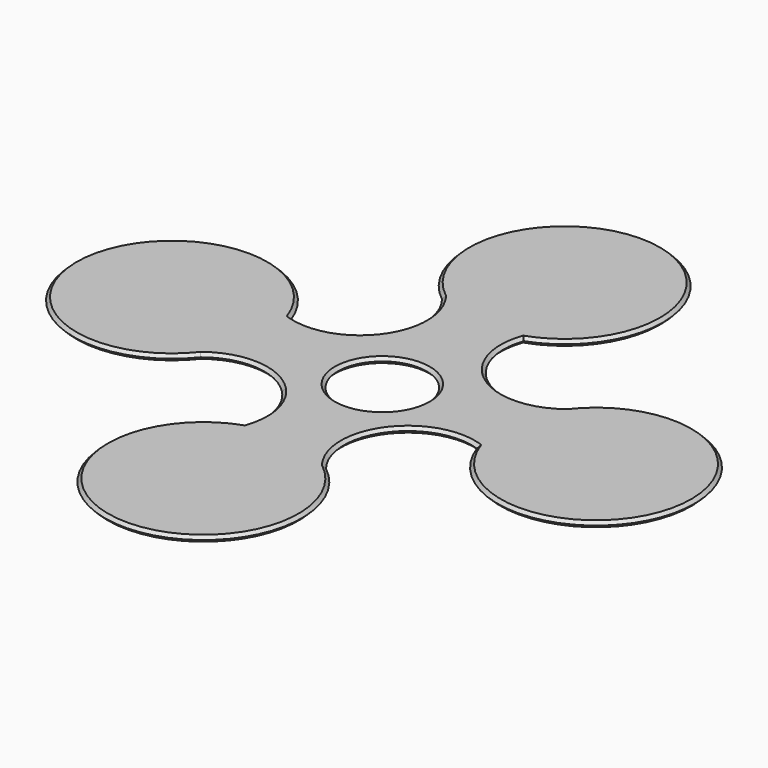
from build123d import *

# Parameters (mm, degrees)
F0_R        = 3.6516934022
F1_DEPTH    = 0.508
F2_C1_SIZE  = 0.254
F2_C2_SIZE  = 0.2539
F2_C3_SIZE  = 0.254
F2_C4_SIZE  = 0.2539
F2_C5_SIZE  = 0.254
F2_C6_SIZE  = 0.2539
F2_C7_SIZE  = 0.254
F2_C8_SIZE  = 0.2539
F2_C9_SIZE  = 0.2539
F2_C10_SIZE = 0.2536
F2_C11_SIZE = 0.254
F2_C12_SIZE = 0.2539
F2_C13_SIZE = 0.2539
F2_C14_SIZE = 0.2536
F2_C15_SIZE = 0.2539
F2_C16_SIZE = 0.2536
F2_C17_SIZE = 0.2539
F2_C18_SIZE = 0.2536


# Not quite as in the source:
# - a fillet or chamfer is up to 0.001 mm smaller than in the source, because OpenCascade refuses the exact size


with BuildPart() as f1:
    # F0 (on Top) → F1 (new body)
    with BuildSketch(Plane.XY):
        with BuildLine():
            ThreePointArc((-4.6809479161, -4.4692134998), (-4.2851428425, -4.9358337251), (-3.9462508024, -5.445292532))
            ThreePointArc((-3.9462508024, -5.445292532), (-3.2543970352, -7.5756381968), (-3.5123975908, -9.8006033651))
            ThreePointArc((-3.5123975908, -9.8006033651), (0.5657181683, -9.1143610896), (4.2157772611, -11.0583325976))
            ThreePointArc((4.2157772611, -11.0583325976), (4.0349146255, -4.7562355253), (10.0331924761, -2.8146378249))
            ThreePointArc((10.0331924761, -2.8146378249), (9.3469502005, 1.2634779342), (11.2909217086, 4.913537027))
            ThreePointArc((11.2909217086, 4.913537027), (7.9764094343, 3.7712610201), (4.6809479161, 4.9673878837))
            ThreePointArc((4.6809479161, 4.9673878837), (4.4188770442, 5.1978976137), (4.1726827472, 5.445292532))
            ThreePointArc((4.1726827472, 5.445292532), (2.8785820733, 7.9323939108), (3.0472269358, 10.730952242))
            ThreePointArc((3.0472269358, 10.730952242), (-1.0308888232, 10.0447099664), (-4.6809479161, 11.9886814745))
            ThreePointArc((-4.6809479161, 11.9886814745), (-4.5000852805, 5.6865844021), (-10.498363131, 3.7449867017))
            ThreePointArc((-10.498363131, 3.7449867017), (-9.8121208555, -0.3331290573), (-11.7560923635, -3.9831881502))
            ThreePointArc((-11.7560923635, -3.9831881502), (-8.1241949781, -2.8530951946), (-4.6809479161, -4.4692134998))
        make_face()
        Circle(F0_R, mode=Mode.SUBTRACT)
        with BuildLine():
            ThreePointArc((-10.498363131, 3.7449867017), (-26.1092040598, 2.319155388), (-11.7560923635, -3.9831881502))
            ThreePointArc((-11.7560923635, -3.9831881502), (-9.8121208555, -0.3331290573), (-10.498363131, 3.7449867017))
        make_face()
        with BuildLine():
            ThreePointArc((4.2157772611, -11.0583325976), (0.5657181683, -9.1143610896), (-3.5123975908, -9.8006033651))
            ThreePointArc((-3.5123975908, -9.8006033651), (-2.0865662771, -25.4114442939), (4.2157772611, -11.0583325976))
        make_face()
        with BuildLine():
            ThreePointArc((11.2909217086, 4.913537027), (9.3469502005, 1.2634779342), (10.0331924761, -2.8146378249))
            ThreePointArc((10.0331924761, -2.8146378249), (25.6440334048, -1.3888065112), (11.2909217086, 4.913537027))
        make_face()
        with BuildLine():
            ThreePointArc((3.0472269358, 10.730952242), (1.6213956221, 26.3417931707), (-4.6809479161, 11.9886814745))
            ThreePointArc((-4.6809479161, 11.9886814745), (-1.0308888232, 10.0447099664), (3.0472269358, 10.730952242))
        make_face()
    extrude(amount=F1_DEPTH)

    # F2: chamfer of 0.254 on 18 edges, made by hand

    # F2_c1
    f2_c1_edges = [f1.edges().sort_by_distance(p)[0] for p in [
        (-5.4539952912, -3.8023255146, 0),
    ]]
    chamfer(f2_c1_edges, length=F2_C1_SIZE)

    # F2_c2 (size 0.254 in the source; OpenCascade refuses exactly that, so slightly less here)
    f2_c2_edges = [f1.edges().sort_by_distance(p)[0] for p in [
        (-5.4539952912, -3.8023255146, 0.508),
    ]]
    chamfer(f2_c2_edges, length=F2_C2_SIZE)

    # F2_c3
    f2_c3_edges = [f1.edges().sort_by_distance(p)[0] for p in [
        (4.0349146255, -4.7562355253, 0),
    ]]
    chamfer(f2_c3_edges, length=F2_C3_SIZE)

    # F2_c4 (size 0.254 in the source; OpenCascade refuses exactly that, so slightly less here)
    f2_c4_edges = [f1.edges().sort_by_distance(p)[0] for p in [
        (4.0349146255, -4.7562355253, 0.508),
    ]]
    chamfer(f2_c4_edges, length=F2_C4_SIZE)

    # F2_c5
    f2_c5_edges = [f1.edges().sort_by_distance(p)[0] for p in [
        (4.9888246362, 4.7326743914, 0),
    ]]
    chamfer(f2_c5_edges, length=F2_C5_SIZE)

    # F2_c6 (size 0.254 in the source; OpenCascade refuses exactly that, so slightly less here)
    f2_c6_edges = [f1.edges().sort_by_distance(p)[0] for p in [
        (4.9888246362, 4.7326743914, 0.508),
    ]]
    chamfer(f2_c6_edges, length=F2_C6_SIZE)

    # F2_c7
    f2_c7_edges = [f1.edges().sort_by_distance(p)[0] for p in [
        (-4.5000852805, 5.6865844021, 0),
    ]]
    chamfer(f2_c7_edges, length=F2_C7_SIZE)

    # F2_c8 (size 0.254 in the source; OpenCascade refuses exactly that, so slightly less here)
    f2_c8_edges = [f1.edges().sort_by_distance(p)[0] for p in [
        (-4.5000852805, 5.6865844021, 0.508),
    ]]
    chamfer(f2_c8_edges, length=F2_C8_SIZE)

    # F2_c9 (size 0.254 in the source; OpenCascade refuses exactly that, so slightly less here)
    f2_c9_edges = [f1.edges().sort_by_distance(p)[0] for p in [
        (-26.1092040598, 2.319155388, 0),
    ]]
    chamfer(f2_c9_edges, length=F2_C9_SIZE)

    # F2_c10 (size 0.254 in the source; OpenCascade refuses exactly that, so slightly less here)
    f2_c10_edges = [f1.edges().sort_by_distance(p)[0] for p in [
        (-26.1092040598, 2.319155388, 0.508),
    ]]
    chamfer(f2_c10_edges, length=F2_C10_SIZE)

    # F2_c11
    f2_c11_edges = [f1.edges().sort_by_distance(p)[0] for p in [
        (-3.6516934022, 0, 0),
    ]]
    chamfer(f2_c11_edges, length=F2_C11_SIZE)

    # F2_c12 (size 0.254 in the source; OpenCascade refuses exactly that, so slightly less here)
    f2_c12_edges = [f1.edges().sort_by_distance(p)[0] for p in [
        (-3.6516934022, 0, 0.508),
    ]]
    chamfer(f2_c12_edges, length=F2_C12_SIZE)

    # F2_c13 (size 0.254 in the source; OpenCascade refuses exactly that, so slightly less here)
    f2_c13_edges = [f1.edges().sort_by_distance(p)[0] for p in [
        (-2.0865662771, -25.4114442939, 0),
    ]]
    chamfer(f2_c13_edges, length=F2_C13_SIZE)

    # F2_c14 (size 0.254 in the source; OpenCascade refuses exactly that, so slightly less here)
    f2_c14_edges = [f1.edges().sort_by_distance(p)[0] for p in [
        (-2.0865662771, -25.4114442939, 0.508),
    ]]
    chamfer(f2_c14_edges, length=F2_C14_SIZE)

    # F2_c15 (size 0.254 in the source; OpenCascade refuses exactly that, so slightly less here)
    f2_c15_edges = [f1.edges().sort_by_distance(p)[0] for p in [
        (25.6440334048, -1.3888065112, 0),
    ]]
    chamfer(f2_c15_edges, length=F2_C15_SIZE)

    # F2_c16 (size 0.254 in the source; OpenCascade refuses exactly that, so slightly less here)
    f2_c16_edges = [f1.edges().sort_by_distance(p)[0] for p in [
        (25.6440334048, -1.3888065112, 0.508),
    ]]
    chamfer(f2_c16_edges, length=F2_C16_SIZE)

    # F2_c17 (size 0.254 in the source; OpenCascade refuses exactly that, so slightly less here)
    f2_c17_edges = [f1.edges().sort_by_distance(p)[0] for p in [
        (1.6213956221, 26.3417931707, 0),
    ]]
    chamfer(f2_c17_edges, length=F2_C17_SIZE)

    # F2_c18 (size 0.254 in the source; OpenCascade refuses exactly that, so slightly less here)
    f2_c18_edges = [f1.edges().sort_by_distance(p)[0] for p in [
        (1.6213956221, 26.3417931707, 0.508),
    ]]
    chamfer(f2_c18_edges, length=F2_C18_SIZE)


solid = f1.part
